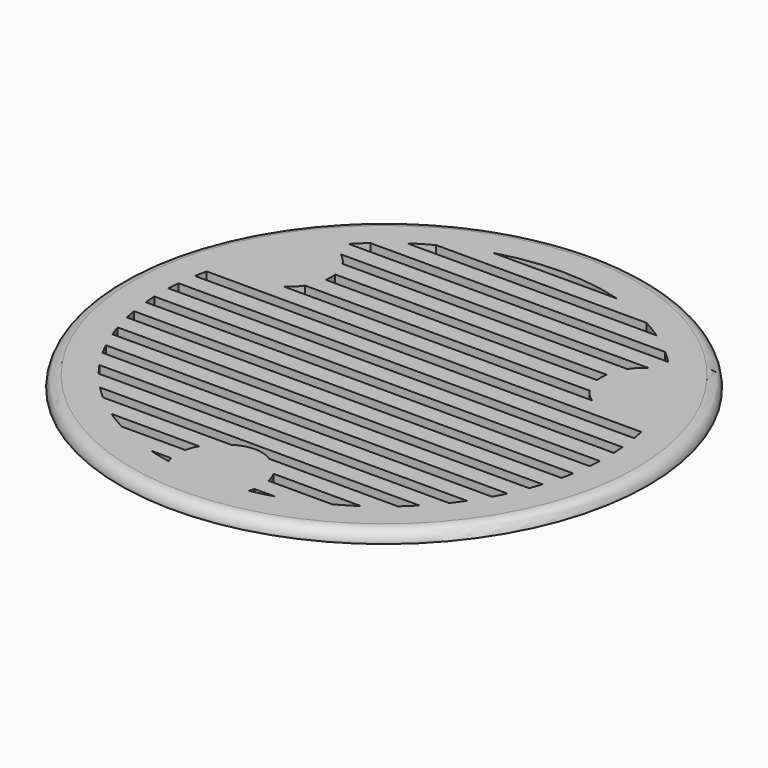
from build123d import *

# Parameters (mm, degrees)
F0_R     = 45
F1_DEPTH = 2
F2_R     = 5.25
F3_DEPTH = 1
F4_R     = 3.25
F5_DEPTH = 5
F6_R     = 2
F7_R     = 1.99999
F9_DEPTH = 25


# Not quite as in the source:
# - a fillet or chamfer is up to 0.001 mm smaller than in the source, because OpenCascade refuses the exact size


with BuildPart() as f1:
    # F0 (on Top) → F1 (new body)
    with BuildSketch(Plane.XY):
        Circle(F0_R)
    extrude(amount=F1_DEPTH)

    # F2 (on face) → F3 (cut)
    with BuildSketch(Plane(origin=(0, 0, 0), x_dir=(1, 0, 0), z_dir=(0, 0, -1))):
        with Locations((0, 35)):
            Circle(F2_R)
        with Locations((-30.3108891325, -17.5)):
            Circle(F2_R)
        with Locations((30.3108891325, -17.5)):
            Circle(F2_R)
    extrude(amount=-F3_DEPTH, mode=Mode.SUBTRACT)

    # F4 (on face) → F5 (join)
    with BuildSketch(Plane(origin=(0, 0, 1), x_dir=(1, 0, 0), z_dir=(0, 0, -1))):
        with Locations((0, 35)):
            Circle(F4_R)
        with Locations((30.3108891325, -17.5)):
            Circle(F4_R)
        with Locations((-30.3108891325, -17.5)):
            Circle(F4_R)
    extrude(amount=F5_DEPTH)

    # F6
    f6_edges = [f1.edges().sort_by_distance(p)[0] for p in [
        (-33.560889, 17.5, -4),
        (-3.25, -35, -4),
        (27.060889, 17.5, -4),
    ]]
    fillet(f6_edges, radius=F6_R)

    # F7 (radius 2 in the source; OpenCascade refuses exactly that, so slightly less here)
    f7_edges = [f1.edges().sort_by_distance(p)[0] for p in [
        (-45, 0, 2),
    ]]
    fillet(f7_edges, radius=F7_R)

    # F8 (on face) → F9 (cut)
    with BuildSketch(Plane.XY.offset(2)):
        with BuildLine():
            Line((17.9373911147, 33.5), (-17.9373911147, 33.5))
            ThreePointArc((-17.9373911147, 33.5), (-19.6214001606, 32.5422902657), (-21.2544113068, 31.5))
            Line((-21.2544113068, 31.5), (21.2544113068, 31.5))
            ThreePointArc((21.2544113068, 31.5), (19.6214001606, 32.5422902657), (17.9373911147, 33.5))
        make_face()
        with BuildLine():
            Line((-7.0931304796, -36.5), (-10.5711872559, -36.5))
            ThreePointArc((-10.5711872559, -36.5), (-8.7211541333, -36.9856927823), (-6.8490250847, -37.3776785714))
            ThreePointArc((-6.8490250847, -37.3776785714), (-6.9848769039, -36.9426771829), (-7.0931304796, -36.5))
        make_face()
        with BuildLine():
            ThreePointArc((-21.2544113068, -31.5), (-19.6214001606, -32.5422902657), (-17.9373911147, -33.5))
            Line((-17.9373911147, -33.5), (-7.0931304796, -33.5))
            ThreePointArc((-7.0931304796, -33.5), (-6.7951561077, -32.4724807673), (-6.3492125496, -31.5))
            Line((-6.3492125496, -31.5), (-21.2544113068, -31.5))
        make_face()
        with BuildLine():
            ThreePointArc((-27.2350876628, -26.5), (-26.2039506035, -27.5200467436), (-25.1346374551, -28.5))
            Line((-25.1346374551, -28.5), (-3.2113081447, -28.5))
            ThreePointArc((-3.2113081447, -28.5), (0, -27.5), (3.2113081447, -28.5))
            Line((3.2113081447, -28.5), (25.1346374551, -28.5))
            ThreePointArc((25.1346374551, -28.5), (26.2039506035, -27.5200467436), (27.2350876628, -26.5))
            Line((27.2350876628, -26.5), (-27.2350876628, -26.5))
        make_face()
        with BuildLine():
            ThreePointArc((-31.3328900678, -21.5), (-30.6138735789, -22.5120133372), (-29.8621834433, -23.5))
            Line((-29.8621834433, -23.5), (29.8621834433, -23.5))
            ThreePointArc((29.8621834433, -23.5), (30.6138735789, -22.5120133372), (31.3328900678, -21.5))
            Line((31.3328900678, -21.5), (-31.3328900678, -21.5))
        make_face()
        with BuildLine():
            ThreePointArc((-34.2308340535, -16.5), (-33.7265552305, -17.5076975151), (-33.1926196616, -18.5))
            Line((-33.1926196616, -18.5), (33.1926196616, -18.5))
            ThreePointArc((33.1926196616, -18.5), (33.7265552305, -17.5076975151), (34.2308340535, -16.5))
            Line((34.2308340535, -16.5), (-34.2308340535, -16.5))
        make_face()
        with BuildLine():
            ThreePointArc((-36.2180894029, -11.5), (-35.8835416114, -12.5048567133), (-35.5211204778, -13.5))
            Line((-35.5211204778, -13.5), (35.5211204778, -13.5))
            ThreePointArc((35.5211204778, -13.5), (35.8835416114, -12.5048567133), (36.2180894029, -11.5))
            Line((36.2180894029, -11.5), (-36.2180894029, -11.5))
        make_face()
        with BuildLine():
            ThreePointArc((-37.439951923, -6.5), (-37.2519722478, -7.5027037562), (-37.0371435184, -8.5))
            Line((-37.0371435184, -8.5), (37.0371435184, -8.5))
            ThreePointArc((37.0371435184, -8.5), (37.2519722478, -7.5027037562), (37.439951923, -6.5))
            Line((37.439951923, -6.5), (-37.439951923, -6.5))
        make_face()
        with BuildLine():
            ThreePointArc((-37.9703831953, -1.5), (-37.9176166167, -2.5008698704), (-37.838472485, -3.5))
            Line((-37.838472485, -3.5), (37.838472485, -3.5))
            ThreePointArc((37.838472485, -3.5), (37.9176166167, -2.5008698704), (37.9703831953, -1.5))
            Line((37.9703831953, -1.5), (-37.9703831953, -1.5))
        make_face()
        with BuildLine():
            ThreePointArc((-37.838472485, 3.5), (-37.9176166167, 2.5008698704), (-37.9703831953, 1.5))
            Line((-37.9703831953, 1.5), (37.9703831953, 1.5))
            ThreePointArc((37.9703831953, 1.5), (37.9176166167, 2.5008698704), (37.838472485, 3.5))
            Line((37.838472485, 3.5), (-37.838472485, 3.5))
        make_face()
        with BuildLine():
            ThreePointArc((-37.0371435184, 8.5), (-37.2519722478, 7.5027037562), (-37.439951923, 6.5))
            Line((-37.439951923, 6.5), (37.439951923, 6.5))
            ThreePointArc((37.439951923, 6.5), (37.2519722478, 7.5027037562), (37.0371435184, 8.5))
            Line((37.0371435184, 8.5), (-37.0371435184, 8.5))
        make_face()
        with BuildLine():
            Line((24.2641958212, 13.5), (-24.2641958212, 13.5))
            ThreePointArc((-24.2641958212, 13.5), (-25.1547879454, 12.403224495), (-26.2411839834, 11.5))
            Line((-26.2411839834, 11.5), (26.2411839834, 11.5))
            ThreePointArc((26.2411839834, 11.5), (25.1547879454, 12.403224495), (24.2641958212, 13.5))
        make_face()
        with BuildLine():
            ThreePointArc((-23.1301858243, 18.5), (-23.0608891325, 17.5), (-23.1301858243, 16.5))
            Line((-23.1301858243, 16.5), (23.1301858243, 16.5))
            ThreePointArc((23.1301858243, 16.5), (23.0608891325, 17.5), (23.1301858243, 18.5))
            Line((23.1301858243, 18.5), (-23.1301858243, 18.5))
        make_face()
        with BuildLine():
            ThreePointArc((-26.2411839834, 23.5), (-25.1547879454, 22.596775505), (-24.2641958212, 21.5))
            Line((-24.2641958212, 21.5), (24.2641958212, 21.5))
            ThreePointArc((24.2641958212, 21.5), (25.1547879454, 22.596775505), (26.2411839834, 23.5))
            Line((26.2411839834, 23.5), (-26.2411839834, 23.5))
        make_face()
        with BuildLine():
            ThreePointArc((-25.1346374551, 28.5), (-26.2039506035, 27.5200467436), (-27.2350876628, 26.5))
            Line((-27.2350876628, 26.5), (27.2350876628, 26.5))
            ThreePointArc((27.2350876628, 26.5), (26.2039506035, 27.5200467436), (25.1346374551, 28.5))
            Line((25.1346374551, 28.5), (-25.1346374551, 28.5))
        make_face()
        with BuildLine():
            ThreePointArc((10.5711872559, 36.5), (0, 38), (-10.5711872559, 36.5))
            Line((-10.5711872559, 36.5), (10.5711872559, 36.5))
        make_face()
        with BuildLine():
            Line((7.0931304796, -33.5), (17.9373911147, -33.5))
            ThreePointArc((17.9373911147, -33.5), (19.6214001606, -32.5422902657), (21.2544113068, -31.5))
            Line((21.2544113068, -31.5), (6.3492125496, -31.5))
            ThreePointArc((6.3492125496, -31.5), (6.7951561077, -32.4724807673), (7.0931304796, -33.5))
        make_face()
        with BuildLine():
            Line((10.5711872559, -36.5), (7.0931304796, -36.5))
            ThreePointArc((7.0931304796, -36.5), (6.9848769039, -36.9426771829), (6.8490250847, -37.3776785714))
            ThreePointArc((6.8490250847, -37.3776785714), (8.7211541333, -36.9856927823), (10.5711872559, -36.5))
        make_face()
    extrude(amount=-F9_DEPTH, mode=Mode.SUBTRACT)


solid = f1.part
